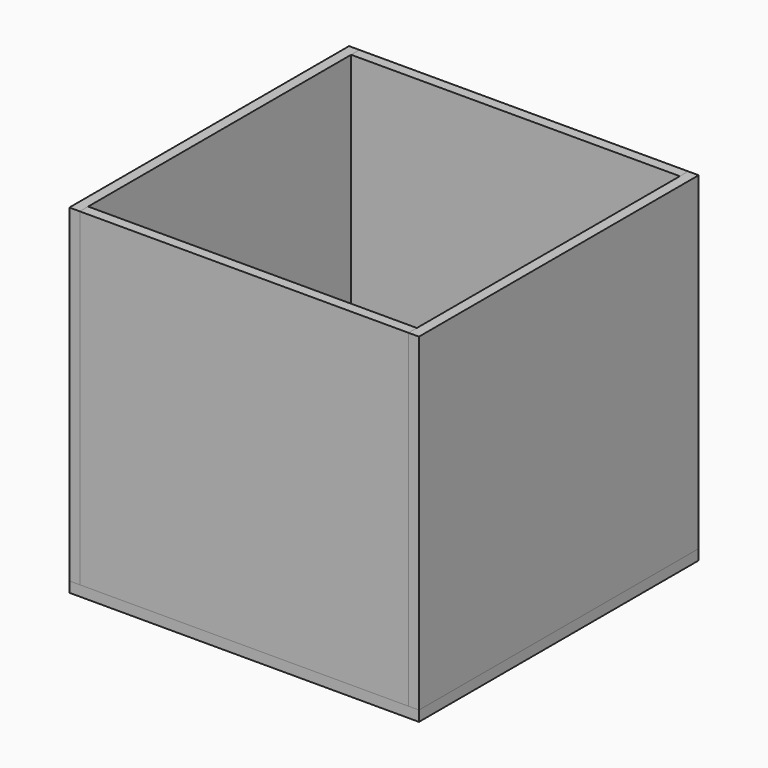
from build123d import *

# Parameters (mm, degrees)
F0_W     = 400
F0_H     = 400
F0_H_2   = 12.7
F1_DEPTH = 12.7
F2_DEPTH = 400
F3_DEPTH = 400
F4_DEPTH = 400
F5_DEPTH = 400


# Not quite as in the source:
# - a length typed as a fraction of an inch, garbled in the dataset ("3 / 203.2 mm" for 3/8 in), is restored


with BuildPart() as f1:
    # F0 (on Top) → F1 (new body)
    with BuildSketch(Plane.XY):
        Rectangle(F0_W, F0_H)
        with Locations((0, -206.35)):
            Rectangle(F0_W, F0_H_2)
        Polygon((200, 212.7), (200, 200), (200, -200), (200, -212.7), (212.7, -212.7), (212.7, 212.7), align=None)
        with Locations((0, 206.35)):
            Rectangle(F0_W, F0_H_2)
        Polygon((-200, -200), (-200, 200), (-200, 212.7), (-212.7, 212.7), (-212.7, -212.7), (-200, -212.7), align=None)
    extrude(amount=-F1_DEPTH)


with BuildPart() as f2:
    # F0 (on Top) → F2 (new body)
    with BuildSketch(Plane.XY):
        Polygon((-200, -200), (-200, 200), (-200, 212.7), (-212.7, 212.7), (-212.7, -212.7), (-200, -212.7), align=None)
    extrude(amount=F2_DEPTH)


with BuildPart() as f3:
    # F0 (on Top) → F3 (new body)
    with BuildSketch(Plane.XY):
        with Locations((0, 206.35)):
            Rectangle(F0_W, F0_H_2)
    extrude(amount=F3_DEPTH)


with BuildPart() as f4:
    # F0 (on Top) → F4 (new body)
    with BuildSketch(Plane.XY):
        Polygon((200, 212.7), (200, 200), (200, -200), (200, -212.7), (212.7, -212.7), (212.7, 212.7), align=None)
    extrude(amount=F4_DEPTH)


with BuildPart() as f5:
    # F0 (on Top) → F5 (new body)
    with BuildSketch(Plane.XY):
        with Locations((0, -206.35)):
            Rectangle(F0_W, F0_H_2)
    extrude(amount=F5_DEPTH)


solid = Compound([f1.part, f2.part, f3.part, f4.part, f5.part])
